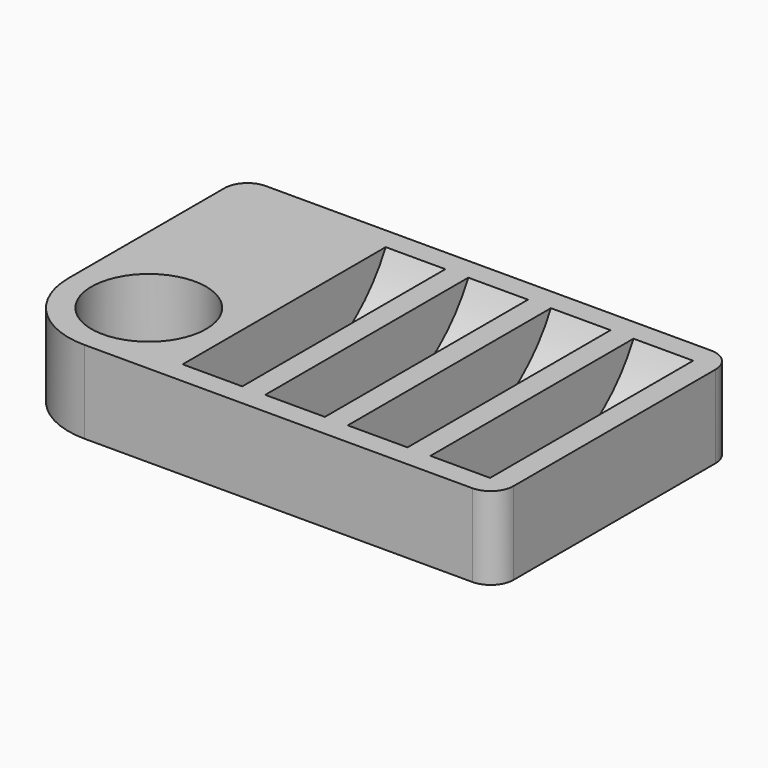
from build123d import *

# Parameters (mm, degrees)
F0_R         = 12.5
F1_DEPTH     = 32
F2_W         = 13
F2_H         = 31
F4_W         = 108.9288368821
F4_H         = 18.1096374691
F5_DEPTH     = 65.001
F6_TEXT_SIZE = 5.5555555556
F7_DEPTH     = 1


# Not quite as in the source:
# - Text() gives the source's letters only with a copy of the font that has no kerning and outlines rounded to 1/6400 em; it was checked with that copy


with BuildPart() as f1:
    # F0 (on Top) → F1 (new body)
    with BuildSketch(Plane.XY):
        with BuildLine():
            ThreePointArc((0, 17.5), (5.1256313292, 5.1256313292), (17.5, 0))
            Line((17.5, 0), (102, 0))
            ThreePointArc((102, 0), (105.5355339059, 1.4644660941), (107, 5))
            Line((107, 5), (107, 60))
            ThreePointArc((107, 60), (105.5355339059, 63.5355339059), (102, 65))
            Line((102, 65), (5, 65))
            ThreePointArc((5, 65), (1.4644660941, 63.5355339059), (0, 60))
            Line((0, 60), (0, 17.5))
        make_face()
        with Locations((17.5, 17.5)):
            Circle(F0_R, mode=Mode.SUBTRACT)
    extrude(amount=F1_DEPTH)

    # F2 (on face) → F3 (revolve, cut)
    with BuildSketch(Plane.XY.offset(32)):
        with Locations((41.5, 17)):
            Rectangle(F2_W, F2_H)
        with Locations((59.5, 17)):
            Rectangle(F2_W, F2_H)
        with Locations((77.5, 17)):
            Rectangle(F2_W, F2_H)
        with Locations((95.5, 17)):
            Rectangle(F2_W, F2_H)
    revolve(axis=Axis((41.5, 32.5, 32), (1, 0, 0)), mode=Mode.SUBTRACT)

    # F4 (on face) → F5 (cut, through all)
    with BuildSketch(Plane.XZ):
        with Locations((54.4644184411, 27.0548187345)):
            Rectangle(F4_W, F4_H)
    extrude(amount=-F5_DEPTH, mode=Mode.SUBTRACT)

    # F6 (on face) → F7 (cut)
    with BuildSketch(Plane(origin=(0, 0, 0), x_dir=(1, 0, 0), z_dir=(0, 0, -1))):
        with Locations((30, -9)):
            Text('865', F6_TEXT_SIZE, font='Open Sans', text_align=(TextAlign.LEFT, TextAlign.BOTTOM))
    extrude(amount=-F7_DEPTH, mode=Mode.SUBTRACT)


solid = f1.part
